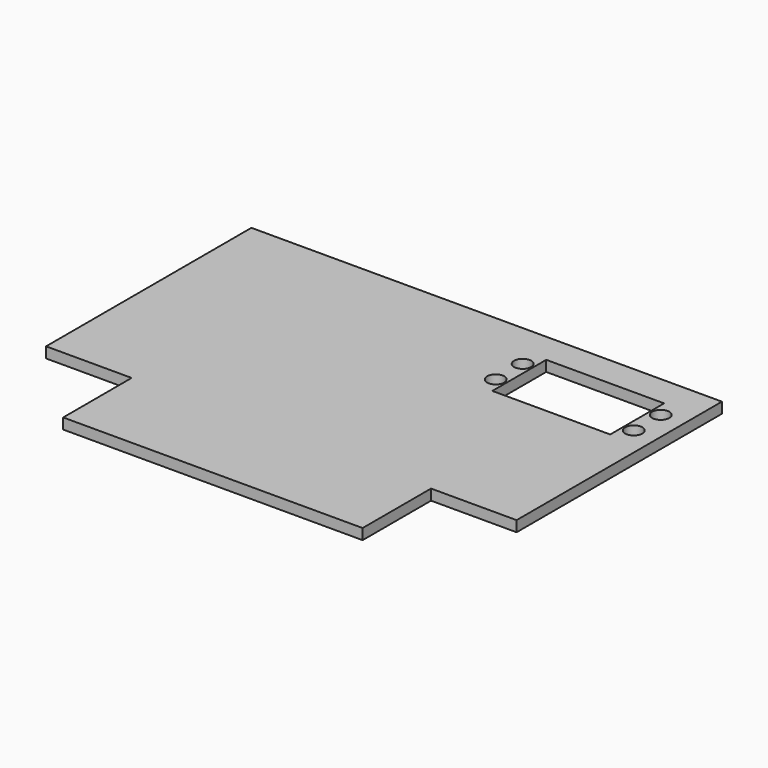
from build123d import *

# Parameters (mm, degrees)
F0_R     = 2.54
F1_DEPTH = 3.175


# Not quite as in the source:
# - a length typed as a fraction of an inch, garbled in the dataset ("3 / 203.2 mm" for 3/8 in), is restored


with BuildPart() as f1:
    # F0 (on Top) → F1 (new body)
    with BuildSketch(Plane.XY):
        Polygon((139.7, 101.6), (0, 101.6), (0, 25.4), (25.4, 25.4), (25.4, 0), (114.3, 0), (114.3, 25.4), (139.7, 25.4), align=None)
        with Locations((91.775, 77.55)):
            Circle(F0_R, mode=Mode.SUBTRACT)
        with Locations((91.775, 87.55)):
            Circle(F0_R, mode=Mode.SUBTRACT)
        Polygon((94.775, 92.55), (104.775, 92.55), (129.775, 92.55), (129.775, 72.55), (104.775, 72.55), (94.775, 72.55), align=None, mode=Mode.SUBTRACT)
        with Locations((132.775, 77.55)):
            Circle(F0_R, mode=Mode.SUBTRACT)
        with Locations((132.775, 87.55)):
            Circle(F0_R, mode=Mode.SUBTRACT)
    extrude(amount=F1_DEPTH)


solid = f1.part
